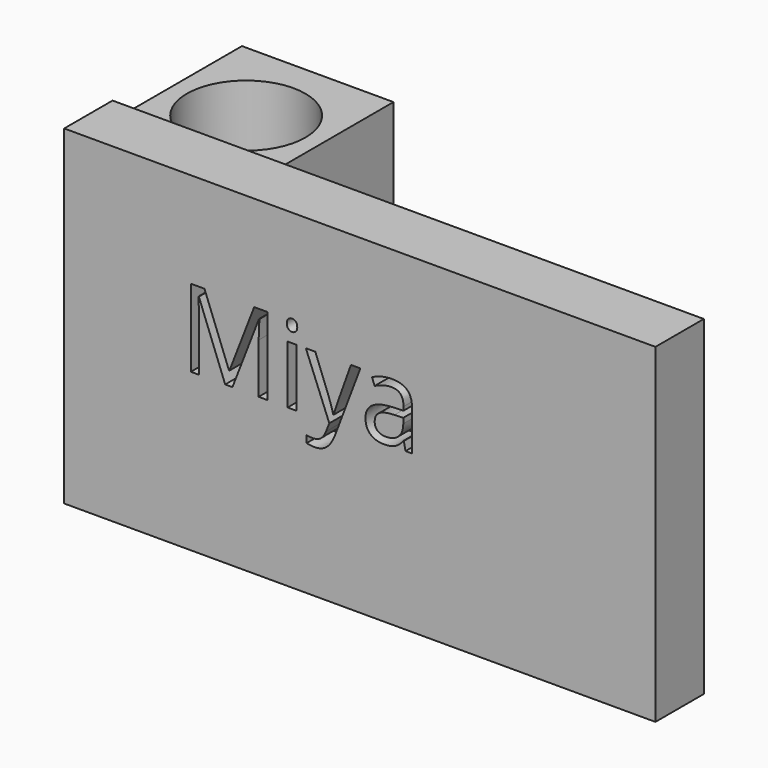
from build123d import *

# Parameters (mm, degrees)
F0_W         = 99.3672609329
F0_H         = 55.4908066988
F1_DEPTH     = 10.16
F2_TEXT_SIZE = 18.2546203076
F3_DEPTH     = 5.08
F4_W         = 25.4651941359
F4_H         = 50.4375156015
F5_DEPTH     = 25.4
F6_R         = 9.9705132225
F7_DEPTH     = 53.6876263555


# Not quite as in the source:
# - Text() gives the source's letters only with a copy of the font that has no kerning and outlines rounded to 1/6400 em; it was checked with that copy


with BuildPart() as f1:
    # F0 (on Front) → F1 (new body)
    with BuildSketch(Plane.XZ):
        with Locations((4.8854015768, 5.4384693503)):
            Rectangle(F0_W, F0_H)
    extrude(amount=F1_DEPTH)

    # F2 (on face) → F3 (cut)
    with BuildSketch(Plane.XZ.offset(10.16)):
        with Locations((-25.3009032458, 4.1072894819)):
            Text('Miya', F2_TEXT_SIZE, font='Open Sans', text_align=(TextAlign.LEFT, TextAlign.BOTTOM))
    extrude(amount=-F3_DEPTH, mode=Mode.SUBTRACT)

    # F4 (on face) → F5 (join)
    with BuildSketch(Plane(origin=(0, 0, 0), x_dir=(-1, 0, 0), z_dir=(0, 1, 0))):
        with Locations((30.640380457, 6.1609344557)):
            Rectangle(F4_W, F4_H)
    extrude(amount=F5_DEPTH)

    # F6 (on face) → F7 (cut, through all)
    with BuildSketch(Plane.XY.offset(31.3796922565)):
        with Locations((-30.6029040366, 10.3238709271)):
            Circle(F6_R)
    extrude(amount=-F7_DEPTH, mode=Mode.SUBTRACT)


solid = f1.part
